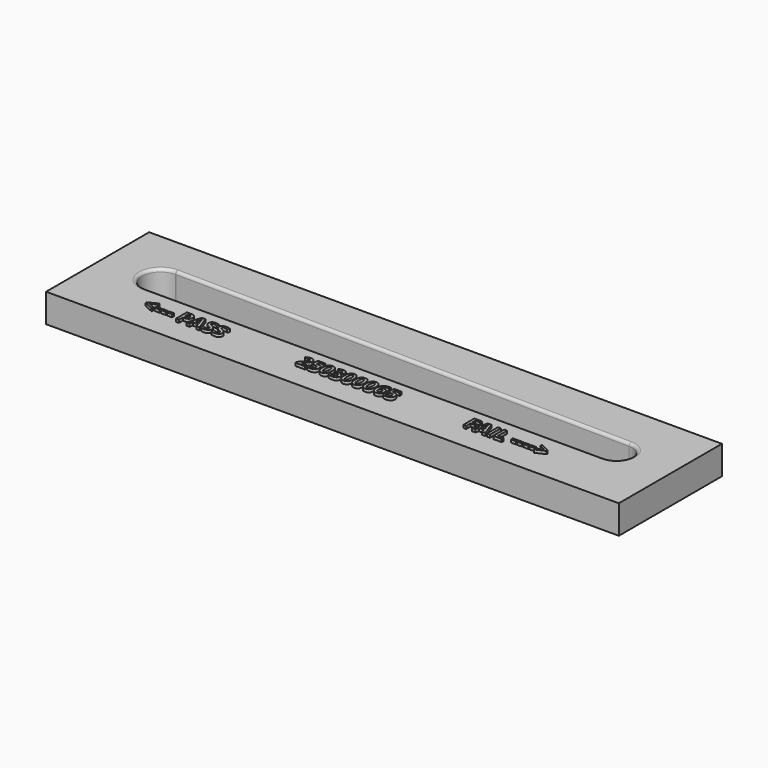
from build123d import *

# Parameters (mm, degrees)
F0_W         = 200
F0_H         = 45
F1_DEPTH     = 10
F2_R         = 1
F3_R         = 1
F4_TEXT_SIZE = 6.6497705929
F5_DEPTH     = 1


# Not quite as in the source:
# - Text() gives the source's letters only with a copy of the font that has no kerning and outlines rounded to 1/6400 em; it was checked with that copy


with BuildPart() as f1:
    # F0 (on Top) → F1 (new body)
    with BuildSketch(Plane.XY):
        with Locations((44.2933450975, 14.2843313776)):
            Rectangle(F0_W, F0_H)
        with BuildLine():
            ThreePointArc((-35.7066549025, 10.2843313776), (-42.2066549025, 16.7843313776), (-35.7066549025, 23.2843313776))
            ThreePointArc((-35.7066549025, 23.2843313776), (-35.6254112494, 23.2838236246), (-35.5441802892, 23.2823004449))
            Line((-35.5441802892, 23.2823004449), (124.2933450975, 21.2843313776))
            ThreePointArc((124.2933450975, 21.2843313776), (129.7933450975, 15.7843313776), (124.2933450975, 10.2843313776))
            Line((124.2933450975, 10.2843313776), (-35.7066549025, 10.2843313776))
        make_face(mode=Mode.SUBTRACT)
    extrude(amount=F1_DEPTH)

    # F2
    f2_edges = [f1.edges().sort_by_distance(p)[0] for p in [
        (44.374582, 22.283316, 10),
        (-42.206655, 16.784331, 10),
        (44.293345, 10.284331, 10),
        (129.793345, 15.784331, 10),
    ]]
    fillet(f2_edges, radius=F2_R)

    # F3
    f3_edges = [f1.edges().sort_by_distance(p)[0] for p in [
        (44.374582, 22.283316, 0),
        (129.793345, 15.784331, 0),
        (44.293345, 10.284331, 0),
    ]]
    fillet(f3_edges, radius=F3_R)

    # F4 (on face) → F5 (join)
    with BuildSketch(Plane.XY.offset(10)):
        with Locations((-29.445162043, 0)):
            Text('<--- PASS               250300065              FAIL ---->', F4_TEXT_SIZE, font='Open Sans', font_style=FontStyle.BOLD, text_align=(TextAlign.LEFT, TextAlign.BOTTOM))
    extrude(amount=F5_DEPTH)


solid = f1.part
